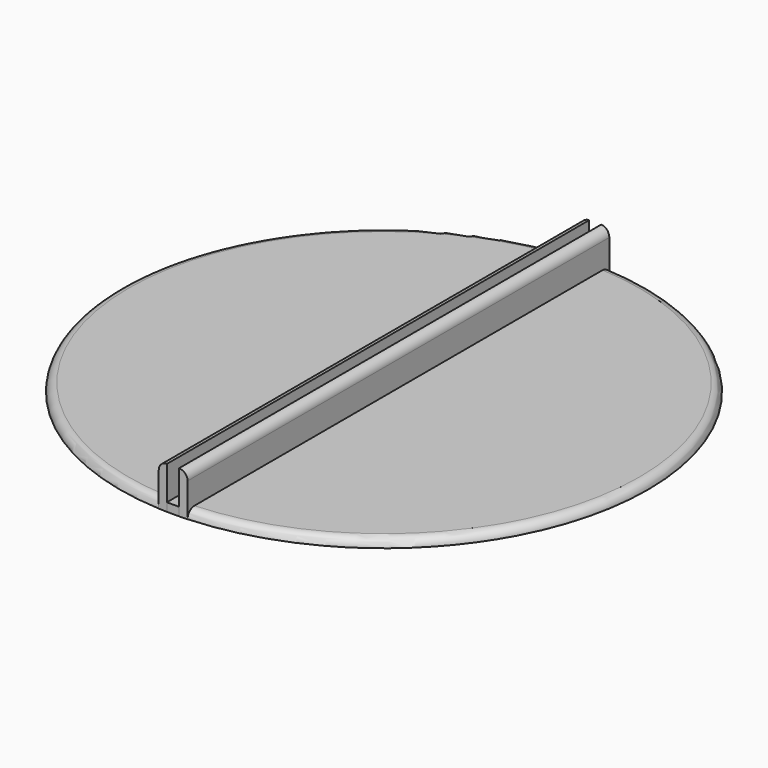
from build123d import *

# Parameters (mm, degrees)
F1_DEPTH      = 1.2
F2_DEPTH      = 6
F3_T2_ANGLE   = 182.9135947962
F3_2_T2_ANGLE = 182.9135947962
F3_3_T1_DEPTH = 80.8878494817
F3_4_T1_DEPTH = 80.8878494817


# Not quite as in the source:
# - a fillet or chamfer that OpenCascade refuses, or shapes differently, is made with other operations: its cross-section is extruded or revolved along the edge and cut away or added


with BuildPart() as f1:
    # F0 (on Top) → F1 (new body)
    with BuildSketch(Plane.XY):
        with BuildLine():
            Line((-2.05, -37.4439247409), (-2.05, 37.4439247409))
            ThreePointArc((-2.05, 37.4439247409), (-37.5, 0), (-2.05, -37.4439247409))
        make_face()
    extrude(amount=F1_DEPTH)

    # F3: fillet of radius 1.2 on 1 edges, made by hand

    # F3_s1 → F3_t2 (revolve, cut)
    with BuildSketch(Plane(origin=(0, 0, 0), x_dir=(0, 0, 1), z_dir=(0.9996767789, -0.0254231717, 0))):
        with BuildLine():
            ThreePointArc((0, -37.5), (0.8485281374, -37.1485281374), (1.2, -36.3))
            Line((1.2, -36.3), (1.2, -37.5))
            Line((1.2, -37.5), (0, -37.5))
        make_face()
    revolve(axis=Axis((0, 0, 1.2), (0, 0, 1)), revolution_arc=F3_T2_ANGLE, mode=Mode.SUBTRACT)


with BuildPart() as f1b:
    # F0 (on Top) → F1, piece 2 (new body)
    with BuildSketch(Plane.XY):
        with BuildLine():
            Line((0.85, -37.490365429), (0.85, 37.490365429))
            ThreePointArc((0.85, 37.490365429), (0, 37.5), (-0.85, 37.490365429))
            Line((-0.85, 37.490365429), (-0.85, -37.490365429))
            ThreePointArc((-0.85, -37.490365429), (0, -37.5), (0.85, -37.490365429))
        make_face()
    extrude(amount=F1_DEPTH)


with BuildPart() as f1c:
    # F0 (on Top) → F1, piece 3 (new body)
    with BuildSketch(Plane.XY):
        with BuildLine():
            ThreePointArc((2.05, -37.4439247409), (27.2316451945, -25.7815340893), (37.5, 0))
            ThreePointArc((37.5, 0), (27.2316451945, 25.7815340893), (2.05, 37.4439247409))
            Line((2.05, 37.4439247409), (2.05, -37.4439247409))
        make_face()
    extrude(amount=F1_DEPTH)

    # F3#2: fillet of radius 1.2 on 1 edges, made by hand

    # F3_2_s1 → F3_2_t2 (revolve, cut)
    with BuildSketch(Plane(origin=(0, 0, 0), x_dir=(0, 0, 1), z_dir=(-0.9996767789, -0.0254231717, 0))):
        with BuildLine():
            ThreePointArc((1.2, 36.3), (0.8485281374, 37.1485281374), (0, 37.5))
            Line((0, 37.5), (1.2, 37.5))
            Line((1.2, 37.5), (1.2, 36.3))
        make_face()
    revolve(axis=Axis((0, 0, 1.2), (0, 0, -1)), revolution_arc=F3_2_T2_ANGLE, mode=Mode.SUBTRACT)


with BuildPart() as f2:
    # F0 (on Top) → F2 (new body)
    with BuildSketch(Plane.XY):
        with BuildLine():
            Line((2.05, -37.4439247409), (2.05, 37.4439247409))
            ThreePointArc((2.05, 37.4439247409), (1.4501859137, 37.4719489861), (0.85, 37.490365429))
            Line((0.85, 37.490365429), (0.85, -37.490365429))
            ThreePointArc((0.85, -37.490365429), (1.4501859137, -37.4719489861), (2.05, -37.4439247409))
        make_face()
    extrude(amount=F2_DEPTH)

    # F3#3: fillet of radius 1.2 on 1 edges, made by hand

    # F3_3_s2 → F3_3_t1 (cut)
    with BuildSketch(Plane.XZ.offset(-40.4439247409)):
        with BuildLine():
            ThreePointArc((2.05, 4.8), (1.6985281374, 5.6485281374), (0.85, 6))
            Line((0.85, 6), (2.05, 6))
            Line((2.05, 6), (2.05, 4.8))
        make_face()
    extrude(amount=F3_3_T1_DEPTH, mode=Mode.SUBTRACT)


with BuildPart() as f2b:
    # F0 (on Top) → F2, piece 2 (new body)
    with BuildSketch(Plane.XY):
        with BuildLine():
            Line((-0.85, -37.490365429), (-0.85, 37.490365429))
            ThreePointArc((-0.85, 37.490365429), (-1.4501859137, 37.4719489861), (-2.05, 37.4439247409))
            Line((-2.05, 37.4439247409), (-2.05, -37.4439247409))
            ThreePointArc((-2.05, -37.4439247409), (-1.4501859137, -37.4719489861), (-0.85, -37.490365429))
        make_face()
    extrude(amount=F2_DEPTH)

    # F3#4: fillet of radius 1.2 on 1 edges, made by hand

    # F3_4_s2 → F3_4_t1 (cut)
    with BuildSketch(Plane.XZ.offset(-40.4439247409)):
        with BuildLine():
            ThreePointArc((-2.05, 4.8), (-1.6985281374, 5.6485281374), (-0.85, 6))
            Line((-0.85, 6), (-2.05, 6))
            Line((-2.05, 6), (-2.05, 4.8))
        make_face()
    extrude(amount=F3_4_T1_DEPTH, mode=Mode.SUBTRACT)


solid = Compound([f1.part, f1b.part, f1c.part, f2.part, f2b.part])
